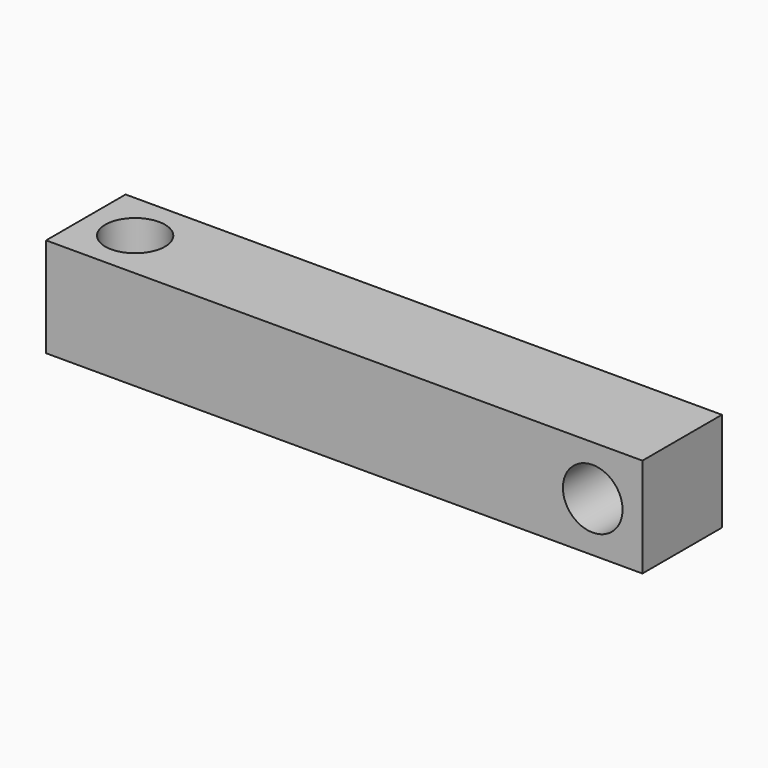
from build123d import *

# Parameters (mm, degrees)
F0_W     = 38.1
F0_H     = 6.35
F0_R     = 1.905
F1_DEPTH = 6.35
F2_R     = 1.905
F3_DEPTH = 6.35


# Not quite as in the source:
# - a feature names something its author has since deleted; it is built from what else it names


with BuildPart() as f1:
    # F0 (on Front) → F1 (new body)
    with BuildSketch(Plane.XZ):
        with Locations((-18.2288356441, -3.7045082716)):
            Rectangle(F0_W, F0_H)
        with Locations((-2.3538356441, -3.7045082716)):
            Circle(F0_R, mode=Mode.SUBTRACT)
    extrude(amount=F1_DEPTH)

    # F2 (on face) → F3 (cut)
    with BuildSketch(Plane.XY.offset(-0.5295082716)):
        with Locations((-34.1285004571, -3.175)):
            Circle(F2_R)
    extrude(amount=-F3_DEPTH, mode=Mode.SUBTRACT)


solid = f1.part
